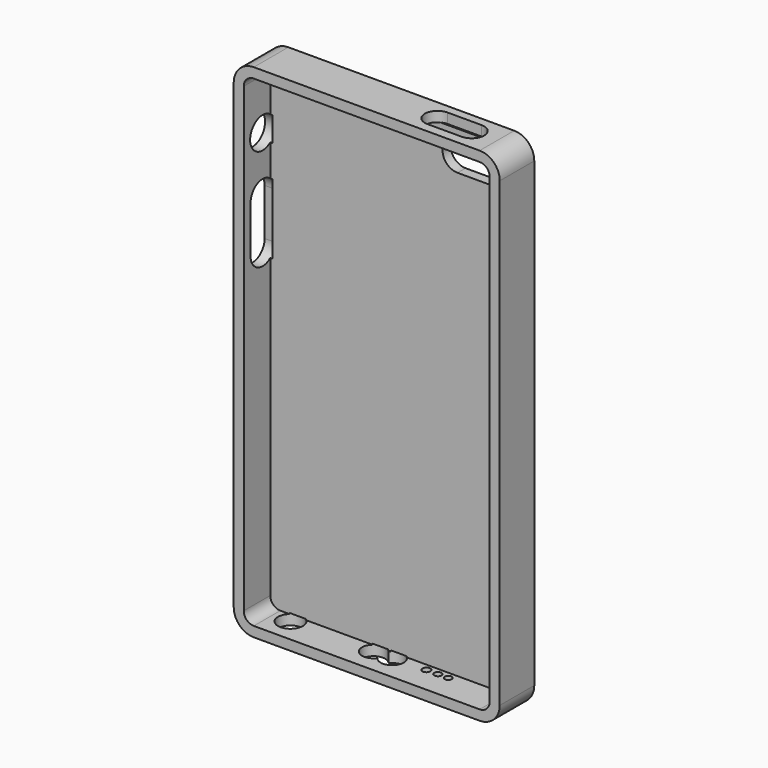
from build123d import *

# Parameters (mm, degrees)
F1_DEPTH  = 10.922
F2_R      = 5.08
F3_T      = -2.54
F5_R      = 0.8828675693
F5_R_2    = 0.9293675191
F5_R_3    = 1.016
F5_R_4    = 3.1543371167
F6_DEPTH  = 2.794
F7_R      = 3.9497200101
F8_DEPTH  = 3.048
F10_DEPTH = 2.54
F11_DEPTH = 25.4
F12_DEPTH = 42.418
F13_DEPTH = 25.4
F14_DEPTH = 2.54


# Not quite as in the source:
# - ends of sketch curves that miss each other by under 0.0002 mm in the source are joined


with BuildPart() as f1:
    # F0 (on Front) → F1 (new body)
    with BuildSketch(Plane.XZ):
        Polygon((32.2100387361, 89.3816531977), (0, 89.3816531977), (-35.0999612639, 89.3816531977), (-35.0999612639, -37.6183468023), (32.2100387361, -37.6183468023), align=None)
    extrude(amount=F1_DEPTH)

    # F2
    f2_edges = [f1.edges().sort_by_distance(p)[0] for p in [
        (-35.099961, -5.461, 89.381653),
        (32.210039, -5.461, 89.381653),
        (32.210039, -5.461, -37.618347),
        (-35.099961, -5.461, -37.618347),
    ]]
    fillet(f2_edges, radius=F2_R)

    # F3
    f3_openings = [f1.faces().sort_by_distance(p)[0] for p in [
        (-1.444961, -10.922, 25.881653),
    ]]
    offset(amount=F3_T, openings=f3_openings)

    # F5 (on face) → F6 (cut)
    with BuildSketch(Plane(origin=(0, 0, -37.6183468023), x_dir=(1, 0, 0), z_dir=(0, 0, -1))):
        with Locations((13.885099197, 4.3037165888)):
            Circle(F5_R)
        with Locations((11.2725288543, 4.3037165888)):
            Circle(F5_R_2)
        with Locations((8.3696719582, 4.3037165888)):
            Circle(F5_R_3)
        with BuildLine():
            ThreePointArc((-2.3474816699, 2.9566967291), (-1.9210459872, 3.7797455945), (-1.7739633397, 4.6949633397))
            ThreePointArc((-1.7739633397, 4.6949633397), (-1.9210459872, 5.6101810849), (-2.3474816699, 6.4332299504))
            ThreePointArc((-2.3474816699, 6.4332299504), (-2.921, 4.6949633397), (-2.3474816699, 2.9566967291))
        make_face()
        with BuildLine():
            ThreePointArc((-2.3474816699, 6.4332299504), (-1.9210459872, 5.6101810849), (-1.7739633397, 4.6949633397))
            ThreePointArc((-1.7739633397, 4.6949633397), (-1.9210459872, 3.7797455945), (-2.3474816699, 2.9566967291))
            ThreePointArc((-2.3474816699, 2.9566967291), (0.9152177452, 1.9210459872), (2.921, 4.6949633397))
            ThreePointArc((2.921, 4.6949633397), (0.9152177452, 7.4688806923), (-2.3474816699, 6.4332299504))
        make_face()
        with BuildLine():
            ThreePointArc((-2.3474816699, 2.9566967291), (-2.921, 4.6949633397), (-2.3474816699, 6.4332299504))
            ThreePointArc((-2.3474816699, 6.4332299504), (-7.6159633397, 4.6949633397), (-2.3474816699, 2.9566967291))
        make_face()
        with Locations((-25.5645439029, 4.8905867152)):
            Circle(F5_R_4)
    extrude(amount=-F6_DEPTH, mode=Mode.SUBTRACT)

    # F7 (on face) → F8 (cut)
    with BuildSketch(Plane(origin=(-35.0999612639, 0, 0), x_dir=(0, -1, 0), z_dir=(-1, 0, 0))):
        with Locations((4.9604894593, 71.5386738494)):
            Circle(F7_R)
        with BuildLine():
            ThreePointArc((1.1504894593, 57.4310126755), (4.9604894593, 53.6210126755), (8.7704894593, 57.4310126755))
            ThreePointArc((8.7704894593, 57.4310126755), (4.9604894593, 61.2410126755), (1.1504894593, 57.4310126755))
        make_face()
        with BuildLine():
            Line((8.7704894593, 45.599225808), (8.7704894593, 57.4310126755))
            ThreePointArc((8.7704894593, 57.4310126755), (4.9604894593, 53.6210126755), (1.1504894593, 57.4310126755))
            Line((1.1504894593, 57.4310126755), (1.1504894593, 45.599225808))
            ThreePointArc((1.1504894593, 45.599225808), (4.9604894593, 49.409225808), (8.7704894593, 45.599225808))
        make_face()
        with BuildLine():
            ThreePointArc((1.1504894593, 45.599225808), (4.9604894593, 41.789225808), (8.7704894593, 45.599225808))
            ThreePointArc((8.7704894593, 45.599225808), (4.9604894593, 49.409225808), (1.1504894593, 45.599225808))
        make_face()
    extrude(amount=-F8_DEPTH, mode=Mode.SUBTRACT)

    # F9 (on face) → F10 (cut)
    with BuildSketch(Plane.XY.offset(89.3816531977)):
        with BuildLine():
            ThreePointArc((20.6356343466, -8.5090005688), (22.8806983769, -7.5790645991), (23.8106343466, -5.3340005688))
            ThreePointArc((23.8106343466, -5.3340005688), (22.8806983769, -3.0889365386), (20.6356343466, -2.1590005688))
            ThreePointArc((20.6356343466, -2.1590005688), (17.4606343466, -5.3340005688), (20.6356343466, -8.5090005688))
        make_face()
        with BuildLine():
            ThreePointArc((20.6356343466, -8.5090005688), (17.4606343466, -5.3340005688), (20.6356343466, -2.1590005688))
            Line((20.6356343466, -2.1590005688), (11.9718069021, -2.1590005688))
            ThreePointArc((11.9718069021, -2.1590005688), (14.2168709324, -3.0889365386), (15.1468069021, -5.3340005688))
            ThreePointArc((15.1468069021, -5.3340005688), (14.2168709324, -7.5790645991), (11.9718069021, -8.5090005688))
            Line((11.9718069021, -8.5090005688), (20.6356343466, -8.5090005688))
        make_face()
        with BuildLine():
            ThreePointArc((15.1468069021, -5.3340005688), (14.2168709324, -3.0889365386), (11.9718069021, -2.1590005688))
            ThreePointArc((11.9718069021, -2.1590005688), (8.7968069021, -5.3340005688), (11.9718069021, -8.5090005688))
            ThreePointArc((11.9718069021, -8.5090005688), (14.2168709324, -7.5790645991), (15.1468069021, -5.3340005688))
        make_face()
    extrude(amount=-F10_DEPTH, mode=Mode.SUBTRACT)

    # F4 (on face) → F11 (join)
    with BuildSketch(Plane.XZ.offset(2.54)):
        with BuildLine():
            ThreePointArc((14.8296833566, 77.0308773467), (17.524812874, 78.1462244598), (18.6413118633, 80.8408769987))
            ThreePointArc((18.6413118633, 80.8408769987), (17.524812874, 83.5355295376), (14.8296833566, 84.6508766507))
            ThreePointArc((14.8296833566, 84.6508766507), (11.0213118633, 80.8408769987), (14.8296833566, 77.0308773467))
        make_face()
        with BuildLine():
            ThreePointArc((23.875676609, 84.6547431762), (20.0634403296, 80.840061919), (23.8773067684, 77.0270104728))
            ThreePointArc((23.8773067684, 77.0270104728), (26.5741176514, 78.1440661157), (27.6911732943, 80.8408769987))
            ThreePointArc((27.6911732943, 80.8408769987), (26.5735412414, 83.5382641685), (23.875676609, 84.6547431762))
        make_face()
        with BuildLine():
            ThreePointArc((14.8296833566, 84.6508766507), (17.524812874, 83.5355295376), (18.6413118633, 80.8408769987))
            ThreePointArc((18.6413118633, 80.8408769987), (17.524812874, 78.1462244598), (14.8296833566, 77.0308773467))
            Line((14.8296833566, 77.0308773467), (23.8773067684, 77.0270101244))
            ThreePointArc((23.8773067684, 77.0270101244), (20.0634403296, 80.840061919), (23.875676609, 84.6547431762))
            Line((23.875676609, 84.6547431762), (14.8296833566, 84.6508766507))
        make_face()
    extrude(amount=F11_DEPTH)

    # F4 (on face) → F12 (cut)
    with BuildSketch(Plane.XZ.offset(2.54)):
        with BuildLine():
            ThreePointArc((14.8296833566, 77.0308773467), (17.524812874, 78.1462244598), (18.6413118633, 80.8408769987))
            ThreePointArc((18.6413118633, 80.8408769987), (17.524812874, 83.5355295376), (14.8296833566, 84.6508766507))
            ThreePointArc((14.8296833566, 84.6508766507), (11.0213118633, 80.8408769987), (14.8296833566, 77.0308773467))
        make_face()
        with BuildLine():
            ThreePointArc((23.875676609, 84.6547431762), (20.0634403296, 80.840061919), (23.8773067684, 77.0270104728))
            ThreePointArc((23.8773067684, 77.0270104728), (26.5741176514, 78.1440661157), (27.6911732943, 80.8408769987))
            ThreePointArc((27.6911732943, 80.8408769987), (26.5735412414, 83.5382641685), (23.875676609, 84.6547431762))
        make_face()
        with BuildLine():
            ThreePointArc((14.8296833566, 84.6508766507), (17.524812874, 83.5355295376), (18.6413118633, 80.8408769987))
            ThreePointArc((18.6413118633, 80.8408769987), (17.524812874, 78.1462244598), (14.8296833566, 77.0308773467))
            Line((14.8296833566, 77.0308773467), (23.8773067684, 77.0270101244))
            ThreePointArc((23.8773067684, 77.0270101244), (20.0634403296, 80.840061919), (23.875676609, 84.6547431762))
            Line((23.875676609, 84.6547431762), (14.8296833566, 84.6508766507))
        make_face()
    extrude(amount=F12_DEPTH, mode=Mode.SUBTRACT)

    # F4 (on face) → F13 (cut)
    with BuildSketch(Plane.XZ.offset(2.54)):
        with BuildLine():
            ThreePointArc((14.8296833566, 77.0308773467), (17.524812874, 78.1462244598), (18.6413118633, 80.8408769987))
            ThreePointArc((18.6413118633, 80.8408769987), (17.524812874, 83.5355295376), (14.8296833566, 84.6508766507))
            ThreePointArc((14.8296833566, 84.6508766507), (11.0213118633, 80.8408769987), (14.8296833566, 77.0308773467))
        make_face()
        with BuildLine():
            ThreePointArc((23.875676609, 84.6547431762), (20.0634403296, 80.840061919), (23.8773067684, 77.0270104728))
            ThreePointArc((23.8773067684, 77.0270104728), (26.5741176514, 78.1440661157), (27.6911732943, 80.8408769987))
            ThreePointArc((27.6911732943, 80.8408769987), (26.5735412414, 83.5382641685), (23.875676609, 84.6547431762))
        make_face()
        with BuildLine():
            ThreePointArc((14.8296833566, 84.6508766507), (17.524812874, 83.5355295376), (18.6413118633, 80.8408769987))
            ThreePointArc((18.6413118633, 80.8408769987), (17.524812874, 78.1462244598), (14.8296833566, 77.0308773467))
            Line((14.8296833566, 77.0308773467), (23.8773067684, 77.0270101244))
            ThreePointArc((23.8773067684, 77.0270101244), (20.0634403296, 80.840061919), (23.875676609, 84.6547431762))
            Line((23.875676609, 84.6547431762), (14.8296833566, 84.6508766507))
        make_face()
    extrude(amount=-F13_DEPTH, mode=Mode.SUBTRACT)

    # F9 (on face) → F14 (cut)
    with BuildSketch(Plane.XY.offset(89.3816531977)):
        with BuildLine():
            ThreePointArc((20.6356343466, -8.5090005688), (22.8806983769, -7.5790645991), (23.8106343466, -5.3340005688))
            ThreePointArc((23.8106343466, -5.3340005688), (22.8806983769, -3.0889365386), (20.6356343466, -2.1590005688))
            ThreePointArc((20.6356343466, -2.1590005688), (17.4606343466, -5.3340005688), (20.6356343466, -8.5090005688))
        make_face()
        with BuildLine():
            ThreePointArc((20.6356343466, -8.5090005688), (17.4606343466, -5.3340005688), (20.6356343466, -2.1590005688))
            Line((20.6356343466, -2.1590005688), (11.9718069021, -2.1590005688))
            ThreePointArc((11.9718069021, -2.1590005688), (14.2168709324, -3.0889365386), (15.1468069021, -5.3340005688))
            ThreePointArc((15.1468069021, -5.3340005688), (14.2168709324, -7.5790645991), (11.9718069021, -8.5090005688))
            Line((11.9718069021, -8.5090005688), (20.6356343466, -8.5090005688))
        make_face()
        with BuildLine():
            ThreePointArc((15.1468069021, -5.3340005688), (14.2168709324, -3.0889365386), (11.9718069021, -2.1590005688))
            ThreePointArc((11.9718069021, -2.1590005688), (8.7968069021, -5.3340005688), (11.9718069021, -8.5090005688))
            ThreePointArc((11.9718069021, -8.5090005688), (14.2168709324, -7.5790645991), (15.1468069021, -5.3340005688))
        make_face()
    extrude(amount=-F14_DEPTH, mode=Mode.SUBTRACT)


solid = f1.part
